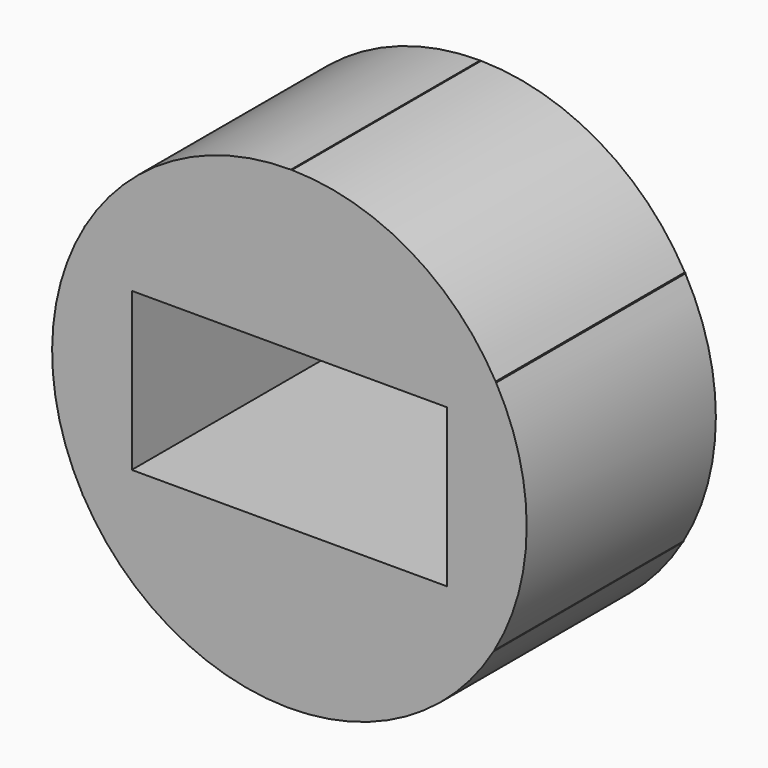
from build123d import *

# Parameters (mm, degrees)
F0_W     = 101.6
F0_H     = 50.8
F1_DEPTH = 38.1


with BuildPart() as f1:
    # F0 (on Front) → F1 (new body, symmetric)
    with BuildSketch(Plane.XZ):
        with BuildLine():
            ThreePointArc((65.9712880145, -38.6489294899), (73.7903692418, -20.0232864477), (76.4588163197, 0))
            ThreePointArc((76.4588163197, 0), (73.9582301549, 19.3940915064), (66.6200350394, 37.5196151947))
            Line((66.6200350394, 37.5196151947), (65.9712880145, -38.6489294899))
        make_face()
        with BuildLine():
            Line((65.9712880145, -38.6489294899), (66.6200350394, 37.5196151947))
            ThreePointArc((66.6200350394, 37.5196151947), (66.5384735192, 37.6640695456), (66.4565987746, 37.808346596))
            Line((66.4565987746, 37.808346596), (0.8170776208, 76.4544503425))
            ThreePointArc((0.8170776208, 76.4544503425), (0.6511957232, 76.4560431695), (0.4853107601, 76.4572760859))
            Line((0.4853107601, 76.4572760859), (-65.8029574185, 38.9348351477))
            ThreePointArc((-65.8029574185, 38.9348351477), (-65.887277796, 38.7919736239), (-65.9712880145, 38.6489294899))
            Line((-65.9712880145, 38.6489294899), (-66.6200350394, -37.5196151947))
            ThreePointArc((-66.6200350394, -37.5196151947), (-66.5384735192, -37.6640695456), (-66.4565987746, -37.808346596))
            Line((-66.4565987746, -37.808346596), (-0.8170776208, -76.4544503425))
            ThreePointArc((-0.8170776208, -76.4544503425), (-0.6511957232, -76.4560431695), (-0.4853107601, -76.4572760859))
            Line((-0.4853107601, -76.4572760859), (65.8029574185, -38.9348351477))
            ThreePointArc((65.8029574185, -38.9348351477), (65.887277796, -38.7919736239), (65.9712880145, -38.6489294899))
        make_face()
        Rectangle(F0_W, F0_H, mode=Mode.SUBTRACT)
        with BuildLine():
            ThreePointArc((66.4565987746, 37.808346596), (66.5384735192, 37.6640695456), (66.6200350394, 37.5196151947))
            Line((66.6200350394, 37.5196151947), (66.6216664831, 37.7111608811))
            Line((66.6216664831, 37.7111608811), (66.4565987746, 37.808346596))
        make_face()
        with BuildLine():
            Line((65.9696565708, -38.8404751763), (65.9712880145, -38.6489294899))
            ThreePointArc((65.9712880145, -38.6489294899), (65.887277796, -38.7919736239), (65.8029574185, -38.9348351477))
            Line((65.8029574185, -38.9348351477), (65.9696565708, -38.8404751763))
        make_face()
        with BuildLine():
            Line((0.8170776208, 76.4544503425), (66.4565987746, 37.808346596))
            ThreePointArc((66.4565987746, 37.808346596), (38.7919736239, 65.887277796), (0.8170776208, 76.4544503425))
        make_face()
        with BuildLine():
            ThreePointArc((-0.4853107601, -76.4572760859), (37.6640695456, -66.5384735192), (65.8029574185, -38.9348351477))
            Line((65.8029574185, -38.9348351477), (-0.4853107601, -76.4572760859))
        make_face()
        with BuildLine():
            ThreePointArc((0.4853107601, 76.4572760859), (0.6511957232, 76.4560431695), (0.8170776208, 76.4544503425))
            Line((0.8170776208, 76.4544503425), (0.6520099123, 76.5516360573))
            Line((0.6520099123, 76.5516360573), (0.4853107601, 76.4572760859))
        make_face()
        with BuildLine():
            Line((-0.6520099123, -76.5516360573), (-0.4853107601, -76.4572760859))
            ThreePointArc((-0.4853107601, -76.4572760859), (-0.6511957232, -76.4560431695), (-0.8170776208, -76.4544503425))
            Line((-0.8170776208, -76.4544503425), (-0.6520099123, -76.5516360573))
        make_face()
        with BuildLine():
            Line((-65.8029574185, 38.9348351477), (0.4853107601, 76.4572760859))
            ThreePointArc((0.4853107601, 76.4572760859), (-37.6640695456, 66.5384735192), (-65.8029574185, 38.9348351477))
        make_face()
        with BuildLine():
            ThreePointArc((-66.4565987746, -37.808346596), (-38.7919736239, -65.887277796), (-0.8170776208, -76.4544503425))
            Line((-0.8170776208, -76.4544503425), (-66.4565987746, -37.808346596))
        make_face()
        with BuildLine():
            ThreePointArc((-65.9712880145, 38.6489294899), (-65.887277796, 38.7919736239), (-65.8029574185, 38.9348351477))
            Line((-65.8029574185, 38.9348351477), (-65.9696565708, 38.8404751763))
            Line((-65.9696565708, 38.8404751763), (-65.9712880145, 38.6489294899))
        make_face()
        with BuildLine():
            Line((-66.6216664831, -37.7111608811), (-66.4565987746, -37.808346596))
            ThreePointArc((-66.4565987746, -37.808346596), (-66.5384735192, -37.6640695456), (-66.6200350394, -37.5196151947))
            Line((-66.6200350394, -37.5196151947), (-66.6216664831, -37.7111608811))
        make_face()
        with BuildLine():
            Line((-66.6200350394, -37.5196151947), (-65.9712880145, 38.6489294899))
            ThreePointArc((-65.9712880145, 38.6489294899), (-76.4560431695, 0.6511957232), (-66.6200350394, -37.5196151947))
        make_face()
    extrude(amount=F1_DEPTH, both=True)


solid = f1.part
